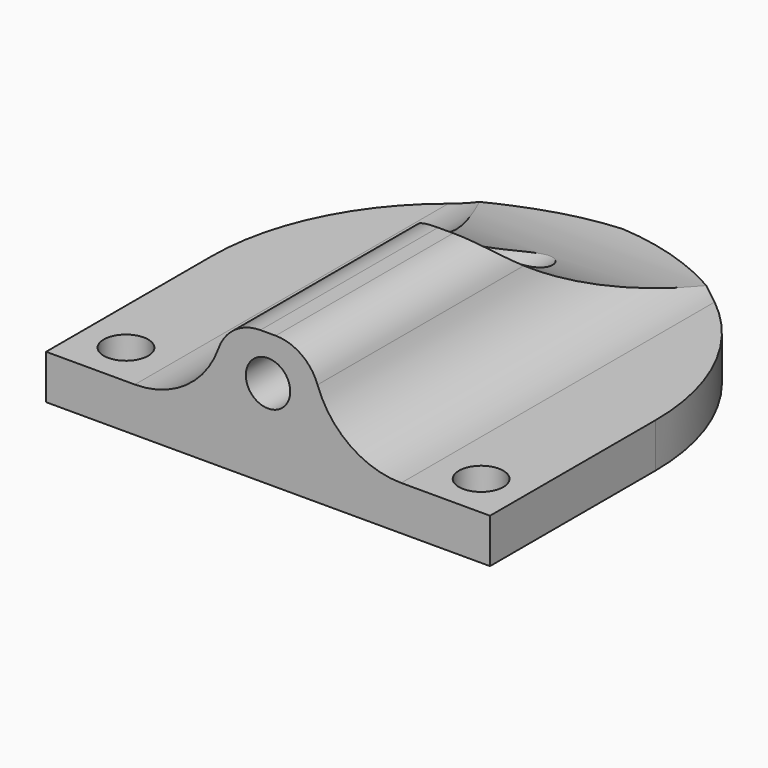
from build123d import *

# Parameters (mm, degrees)
F0_W        = 50
F0_H        = 50
F0_R        = 2.5
F1_DEPTH    = 5
F2_R        = 2.5
F3_DEPTH    = 50
F4_R        = 5
F6_DEPTH    = 50
F7_R        = 3.5
F8_DEPTH    = 23
F9_T1_DEPTH = 138.5987158


# Not quite as in the source:
# - a fillet or chamfer that OpenCascade refuses, or shapes differently, is made with other operations: its cross-section is extruded or revolved along the edge and cut away or added


with BuildPart() as f1:
    # F0 (on Top) → F1 (new body)
    with BuildSketch(Plane.XY):
        Rectangle(F0_W, F0_H)
        with Locations((-20, -20)):
            Circle(F0_R, mode=Mode.SUBTRACT)
        with Locations((20, -20)):
            Circle(F0_R, mode=Mode.SUBTRACT)
    extrude(amount=F1_DEPTH)

    # F2 (on face) → F3 (join, through all)
    with BuildSketch(Plane.XZ.offset(25)):
        with BuildLine():
            Line((-5, 5), (5, 5))
            Line((5, 5), (15, 5))
            ThreePointArc((15, 5), (7.9289321881, 7.9289321881), (5, 15))
            Line((5, 15), (-5, 15))
            ThreePointArc((-5, 15), (-7.9289321881, 7.9289321881), (-15, 5))
            Line((-15, 5), (-5, 5))
        make_face()
        with Locations((0, 10)):
            Circle(F2_R, mode=Mode.SUBTRACT)
    extrude(amount=-F3_DEPTH)

    # F4
    f4_edges = [f1.edges().sort_by_distance(p)[0] for p in [
        (-5, 0, 15),
        (5, 0, 15),
    ]]
    fillet(f4_edges, radius=F4_R)

    # F5 (on face) → F6 (cut, through all)
    with BuildSketch(Plane(origin=(-25, 0, 0), x_dir=(0, -1, 0), z_dir=(-1, 0, 0))):
        with BuildLine():
            Line((-25, 15), (-25, 5))
            ThreePointArc((-25, 5), (-11.5370879822, 7.5927199554), (0, 15))
            Line((0, 15), (-25, 15))
        make_face()
    extrude(amount=-F6_DEPTH, mode=Mode.SUBTRACT)

    # F7 (on face) → F8 (cut)
    with BuildSketch(Plane(origin=(0, 25, 0), x_dir=(-1, 0, 0), z_dir=(0, 1, 0))):
        with Locations((0, 10)):
            Circle(F7_R)
    extrude(amount=-F8_DEPTH, mode=Mode.SUBTRACT)

    # F9: fillet of radius 26.71974316 on 2 edges, made by hand

    # F9_s2 → F9_t1 (cut)
    with BuildSketch(Plane.XY.offset(-66.7993579)):
        with BuildLine():
            ThreePointArc((-1.71974316, 25), (17.17396842, 17.17396842), (25, -1.71974316))
            Line((25, -1.71974316), (25, 25))
            Line((25, 25), (-1.71974316, 25))
        make_face()
        with BuildLine():
            ThreePointArc((1.71974316, 25), (-17.17396842, 17.17396842), (-25, -1.71974316))
            Line((-25, -1.71974316), (-25, 25))
            Line((-25, 25), (1.71974316, 25))
        make_face()
    extrude(amount=F9_T1_DEPTH, mode=Mode.SUBTRACT)


solid = f1.part
